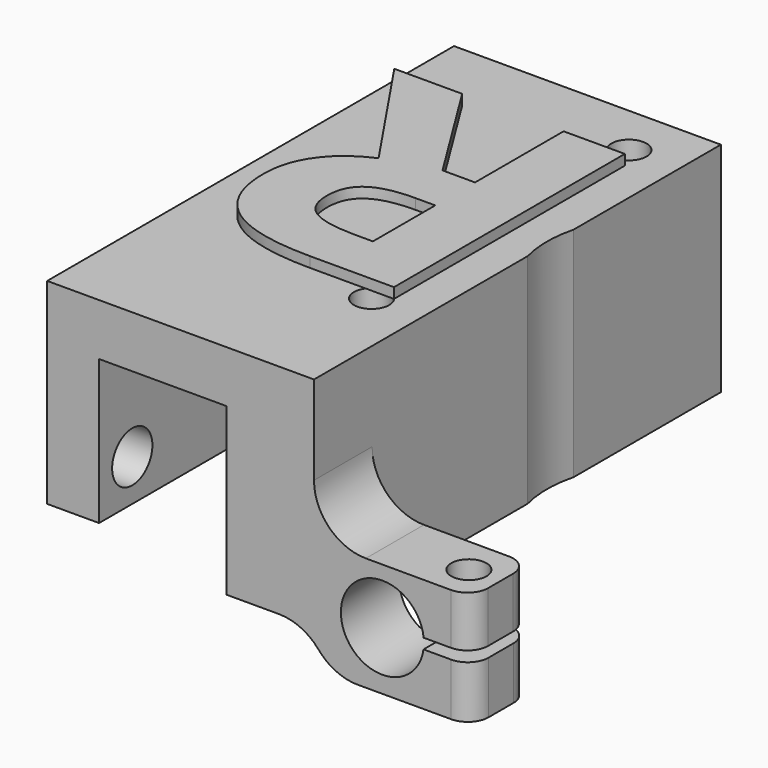
from build123d import *

# Parameters (mm, degrees)
F1_DEPTH      = 7
F2_DEPTH      = 42
F3_R          = 1.7
F3_R_2        = 11
F4_DEPTH      = 21.001
F5_R          = 4
F6_DEPTH      = 10
F7_DEPTH      = 21.001
F8_R          = 1.4
F9_DEPTH      = 11.0209182429
F8_R_2        = 1.7
F10_DEPTH     = 4.9110969969
F11_R         = 5
F12_R         = 5
F13_R         = 5
F14_R         = 2
F15_R         = 2.2
F15_R_2       = 2.4255023423
F16_DEPTH     = 6
F17_TEXT_SIZE = 38.9455612245
F18_DEPTH     = 1


# Not quite as in the source:
# - a feature names something its author has since deleted; it is built from what else it names
# - Text() gives the source's letters only with a copy of the font that has no kerning and outlines rounded to 1/6400 em; it was checked with that copy


with BuildPart() as f1:
    # F0 (on Front) → F1 (new body)
    with BuildSketch(Plane.XZ):
        Polygon((-18.6721007523, 29.8099789735), (-18.6721007523, 10.8925135386), (-13.6721007523, 10.8925135386), (-13.6721007523, 24.8099789735), (-1.3721007523, 24.8099789735), (-1.3721007523, 8.8099789735), (7.0380548998, 8.8099789735), (7.0380548998, 16.2656020473), (7.0380548998, 29.8099789735), align=None)
        Polygon((22.2263195603, 16.2417280634), (7.0380548998, 16.2656020473), (7.0380548998, 8.8099789735), (8.4533044869, 5.2860832236), (22.2553367778, 5.2860832236), (22.2553367778, 10.343908232), (15.5860510706, 10.343908232), (15.5860510706, 11.3388913612), (22.2263195603, 11.3388913612), align=None)
    extrude(amount=F1_DEPTH)

    # F0 (on Front) → F2 (join)
    with BuildSketch(Plane.XZ):
        Polygon((-18.6721007523, 29.8099789735), (-18.6721007523, 10.8925135386), (-13.6721007523, 10.8925135386), (-13.6721007523, 24.8099789735), (-1.3721007523, 24.8099789735), (-1.3721007523, 8.8099789735), (7.0380548998, 8.8099789735), (7.0380548998, 16.2656020473), (7.0380548998, 29.8099789735), align=None)
    extrude(amount=-F2_DEPTH)

    # F3 (on face) → F4 (cut, through all)
    with BuildSketch(Plane(origin=(0, 0, 8.8099789735), x_dir=(1, 0, 0), z_dir=(0, 0, -1))):
        with Locations((2.1850741468, -6)):
            Circle(F3_R)
        with Locations((2.1850741468, -37)):
            Circle(F3_R)
        with Locations((17.6850741468, -21.5)):
            Circle(F3_R_2)
    extrude(amount=-F4_DEPTH, mode=Mode.SUBTRACT)

    # F5 (on face) → F6 (cut)
    with BuildSketch(Plane.XZ.offset(7)):
        with Locations((13.6278992477, 10.8989789735)):
            Circle(F5_R)
    extrude(amount=-F6_DEPTH, mode=Mode.SUBTRACT)

    # F3 (on face) → F7 (cut, through all)
    with BuildSketch(Plane(origin=(0, 0, 8.8099789735), x_dir=(1, 0, 0), z_dir=(0, 0, -1))):
        with Locations((2.1850741468, -6)):
            Circle(F3_R)
        with Locations((2.1850741468, -37)):
            Circle(F3_R)
        with Locations((17.6850741468, -21.5)):
            Circle(F3_R_2)
    extrude(amount=-F7_DEPTH, mode=Mode.SUBTRACT)

    # F8 (on face) → F9 (cut, through all)
    with BuildSketch(Plane(origin=(0.0255847449, 0, 16.2766247417), x_dir=(0.9999987646, 0, -0.0015718685), z_dir=(0.0015718685, 0, 0.9999987646))):
        with Locations((19.2007622419, -3.5767070949)):
            Circle(F8_R)
    extrude(amount=-F9_DEPTH, mode=Mode.SUBTRACT)

    # F8 (on face) → F10 (cut, through all)
    with BuildSketch(Plane(origin=(0.0255847449, 0, 16.2766247417), x_dir=(0.9999987646, 0, -0.0015718685), z_dir=(0.0015718685, 0, 0.9999987646))):
        with Locations((19.2007622419, -3.5767070949)):
            Circle(F8_R_2)
        with Locations((19.2007622419, -3.5767070949)):
            Circle(F8_R, mode=Mode.SUBTRACT)
    extrude(amount=-F10_DEPTH, mode=Mode.SUBTRACT)

    # F11
    f11_edges = [f1.edges().sort_by_distance(p)[0] for p in [
        (7.038055, -3.5, 16.265602),
    ]]
    fillet(f11_edges, radius=F11_R)

    # F12
    f12_edges = [f1.edges().sort_by_distance(p)[0] for p in [
        (7.038055, -3.5, 8.809979),
    ]]
    fillet(f12_edges, radius=F12_R)

    # F13
    f13_edges = [f1.edges().sort_by_distance(p)[0] for p in [
        (8.453304, -3.5, 5.286083),
    ]]
    fillet(f13_edges, radius=F13_R)

    # F14
    f14_edges = [f1.edges().sort_by_distance(p)[0] for p in [
        (22.22632, -7, 13.79031),
        (22.255337, -7, 7.814996),
        (22.22632, 0, 13.79031),
        (22.255337, 0, 7.814996),
    ]]
    fillet(f14_edges, radius=F14_R)

    # F15 (on face) → F16 (cut)
    with BuildSketch(Plane(origin=(-18.6721007523, 0, 0), x_dir=(0, -1, 0), z_dir=(-1, 0, 0))):
        with Locations((-38, 14.8925135386)):
            Circle(F15_R)
        with Locations((3, 14.8925135386)):
            Circle(F15_R_2)
    extrude(amount=-F16_DEPTH, mode=Mode.SUBTRACT)

    # F17 (on face) → F18 (join)
    with BuildSketch(Plane.XY.offset(29.8099789735)):
        with Locations(Location((7.0380548998, 34.8089256118), (0, 0, 180))):
            Text('R', F17_TEXT_SIZE, font='Open Sans', font_style=FontStyle.BOLD, text_align=(TextAlign.LEFT, TextAlign.BOTTOM))
    extrude(amount=F18_DEPTH)


solid = f1.part
